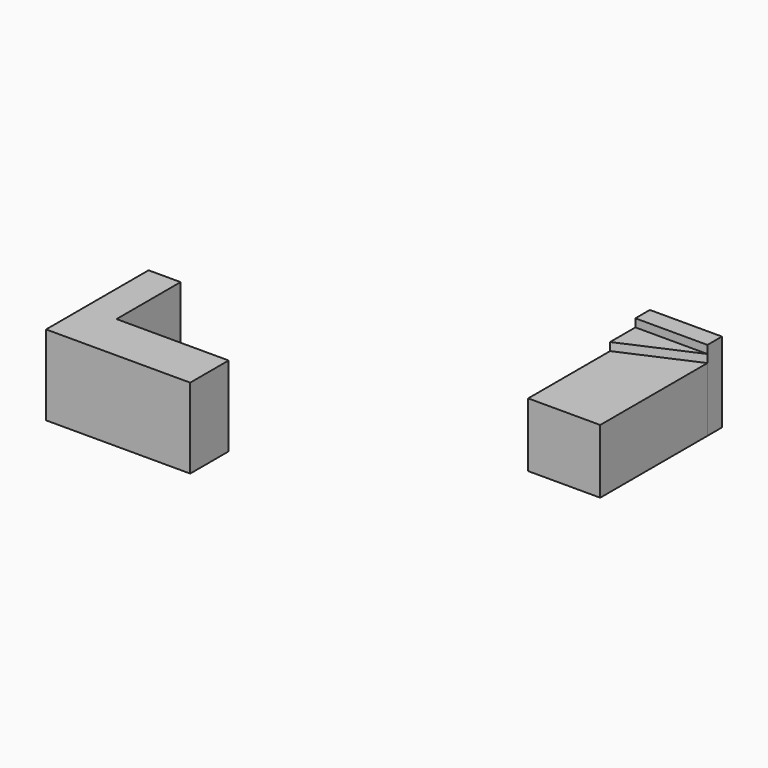
from build123d import *

# Parameters (mm, degrees)
F1_DEPTH = 1000
F0_W     = 900
F0_H     = 226.0670661926
F2_DEPTH = 800
F3_DEPTH = 900


# Not quite as in the source:
# - ends of sketch curves that miss each other by under 0.0002 mm in the source are joined


with BuildPart() as f1:
    # F0 (on Top) → F1 (new body)
    with BuildSketch(Plane.XY):
        Polygon((-3000, -2000), (-1199.9999046326, -2000), (-1199.9999046326, -1399.9999761581), (-2599.9999046326, -1399.9999761581), (-2599.9999046326, -399.9999761581), (-2999.9999046326, -399.9999761581), align=None)
    extrude(amount=F1_DEPTH)


with BuildPart() as f1b:
    # F0 (on Top) → F1, piece 2 (new body)
    with BuildSketch(Plane.XY):
        with Locations((1791.2673473358, 1886.9664669037)):
            Rectangle(F0_W, F0_H)
    extrude(amount=F1_DEPTH)


with BuildPart() as f2:
    # F0 (on Top) → F2 (new body)
    with BuildSketch(Plane.XY):
        Polygon((2241.2673473358, 100), (2241.2673473358, 1773.9329338074), (1341.2673473358, 1378.5252571106), (1341.2673473358, 100), align=None)
    extrude(amount=F2_DEPTH)


with BuildPart() as f3:
    # F0 (on Top) → F3 (new body)
    with BuildSketch(Plane.XY):
        Polygon((1341.2673473358, 1378.5252571106), (2241.2673473358, 1773.9329338074), (1341.2673473358, 1773.9329338074), align=None)
    extrude(amount=F3_DEPTH)


solid = Compound([f1.part, f1b.part, f2.part, f3.part])
